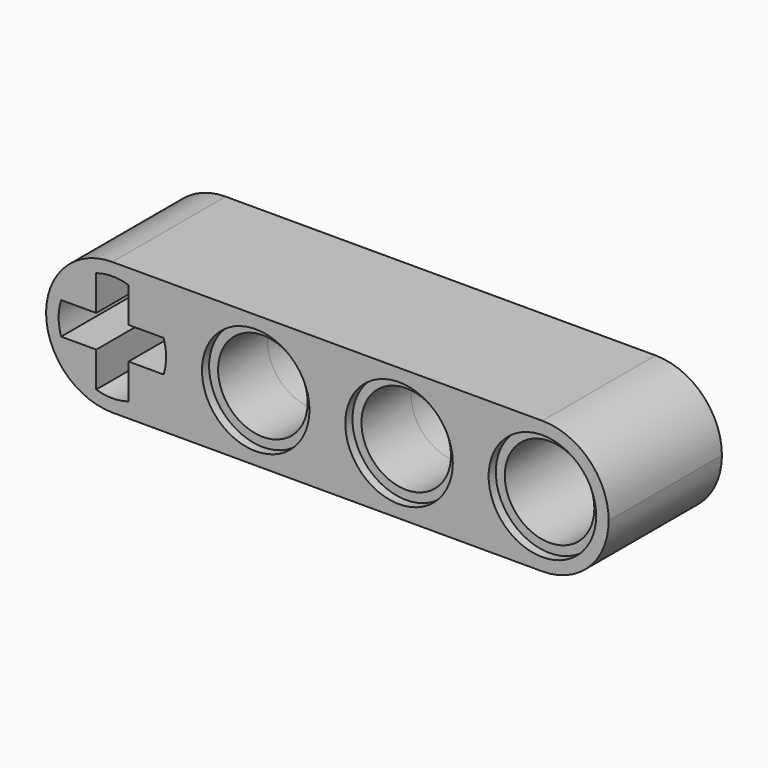
from build123d import *

# Parameters (mm, degrees)
F0_W     = 31.4
F0_H     = 7.4
F0_R     = 3
F1_DEPTH = 3.95
F0_R_2   = 2.499
F2_DEPTH = 3.45
F3_R     = 3.69999


# Not quite as in the source:
# - a fillet or chamfer is up to 0.001 mm smaller than in the source, because OpenCascade refuses the exact size


with BuildPart() as f1:
    # F0 (on Front) → F1 (new body, symmetric)
    with BuildSketch(Plane.XZ):
        Rectangle(F0_W, F0_H)
        with BuildLine():
            ThreePointArc((-12.9, 2.8618176043), (-12, 3), (-11.1, 2.8618176043))
            Line((-11.1, 2.8618176043), (-11.1, 0.9))
            Line((-11.1, 0.9), (-9.1381823957, 0.9))
            ThreePointArc((-9.1381823957, 0.9), (-9, 0), (-9.1381823957, -0.9))
            Line((-9.1381823957, -0.9), (-11.1, -0.9))
            Line((-11.1, -0.9), (-11.1, -2.8618176043))
            ThreePointArc((-11.1, -2.8618176043), (-12, -3), (-12.9, -2.8618176043))
            Line((-12.9, -2.8618176043), (-12.9, -0.9))
            Line((-12.9, -0.9), (-14.8618176043, -0.9))
            ThreePointArc((-14.8618176043, -0.9), (-15, 0), (-14.8618176043, 0.9))
            Line((-14.8618176043, 0.9), (-12.9, 0.9))
            Line((-12.9, 0.9), (-12.9, 2.8618176043))
        make_face(mode=Mode.SUBTRACT)
        with Locations((-4, 0)):
            Circle(F0_R, mode=Mode.SUBTRACT)
        with Locations((4, 0)):
            Circle(F0_R, mode=Mode.SUBTRACT)
        with Locations((12, 0)):
            Circle(F0_R, mode=Mode.SUBTRACT)
    extrude(amount=F1_DEPTH, both=True)

    # F0 (on Front) → F2 (join, symmetric)
    with BuildSketch(Plane.XZ):
        with Locations((-4, 0)):
            Circle(F0_R)
        with Locations((-4, 0)):
            Circle(F0_R_2, mode=Mode.SUBTRACT)
        with Locations((4, 0)):
            Circle(F0_R)
        with Locations((4, 0)):
            Circle(F0_R_2, mode=Mode.SUBTRACT)
        with Locations((12, 0)):
            Circle(F0_R)
        with Locations((12, 0)):
            Circle(F0_R_2, mode=Mode.SUBTRACT)
    extrude(amount=F2_DEPTH, both=True)

    # F3 (radius 3.7 in the source; OpenCascade refuses exactly that, so slightly less here)
    f3_edges = [f1.edges().sort_by_distance(p)[0] for p in [
        (-15.7, 0, 3.7),
        (-15.7, 0, -3.7),
        (15.7, 0, 3.7),
        (15.7, 0, -3.7),
    ]]
    fillet(f3_edges, radius=F3_R)


solid = f1.part
